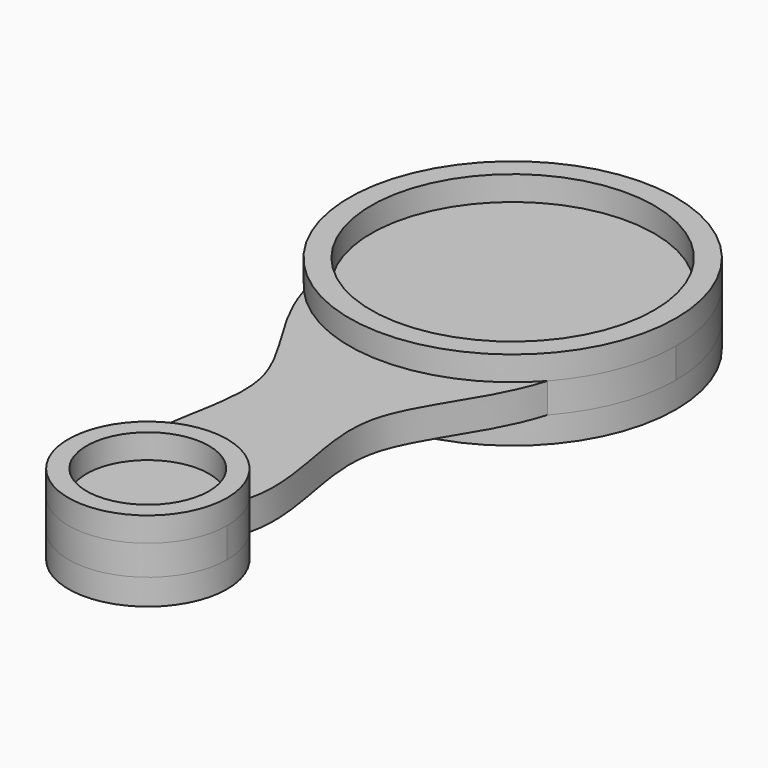
from build123d import *
from build123d import SkipClean  # not in build123d's __all__

# Parameters (mm, degrees)
F1_DEPTH      = 3.3
F2_R          = 18
F2_R_2        = 15.6
F2_R_3        = 8.75
F2_R_4        = 6.75
F3_DEPTH      = 2.85
F3_DEPTH_BACK = 6


with BuildPart() as f1:
    # F0 (on Top) → F1 (new body)
    with BuildSketch(Plane.XY):
        with BuildLine():
            add(Edge.make_bspline(
                [(7.0372224634, -21.05), (8.3671803407, -15.6501668156), (2.1195257428, -2.6023508459), (11.4288521337, 5.4147908541), (13.416407865, 12)],
                knots=[0, 0, 0, 0, 0.4970922674, 1, 1, 1, 1], degree=3))
            ThreePointArc((13.416407865, 12), (0, 42), (-13.416407865, 12))
            add(Edge.make_bspline(
                [(-7.0372224634, -21.05), (-8.3671803407, -15.6501668156), (-2.1195257428, -2.6023508459), (-11.4288521337, 5.4147908541), (-13.416407865, 12)],
                knots=[0, 0, 0, 0, 0.4970922674, 1, 1, 1, 1], degree=3))
            ThreePointArc((-7.0372224634, -21.05), (0, -35), (7.0372224634, -21.05))
        make_face()
    extrude(amount=F1_DEPTH)

    # F2 (on face) → F3 (join, two sides)
    with BuildSketch(Plane(origin=(0, 0, 0), x_dir=(1, 0, 0), z_dir=(0, 0, -1))) as f3_sk:
        with Locations((0, -24)):
            Circle(F2_R)
        with Locations((0, -24)):
            Circle(F2_R_2, mode=Mode.SUBTRACT)
        with Locations((0, 26.25)):
            Circle(F2_R_3)
        with Locations((0, 26.25)):
            Circle(F2_R_4, mode=Mode.SUBTRACT)
    with SkipClean():  # cleaning this boolean's faces spoils the solid; the shape is the same uncleaned
        extrude(amount=F3_DEPTH)
        extrude(f3_sk.sketch, amount=-F3_DEPTH_BACK)


solid = f1.part
